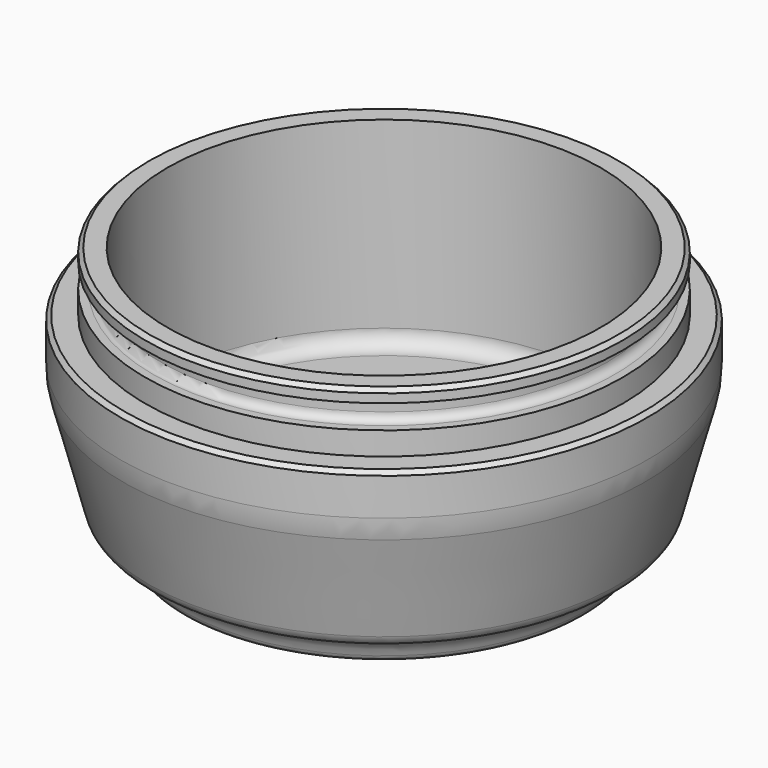
from build123d import *

# Parameters (mm, degrees)
F3_R    = 2
F4_R    = 1
F5_R    = 2
F8_R    = 10
F6_SIZE = 0.5
F9_SIZE = 0.5
F7_R    = 1


# Not quite as in the source:
# - a fillet or chamfer that OpenCascade refuses, or shapes differently, is made with other operations: its cross-section is extruded or revolved along the edge and cut away or added


with BuildPart() as f1:
    # F0 (on Front) → F1 (revolve)
    with BuildSketch(Plane.XZ):
        Polygon((0, -6.6736775178), (-27.25, -6.6736775178), (-27.25, 18.4263224822), (-30.05, 18.4263224822), (-30.05, 16.8263224822), (-28.05, 16.8263224822), (-28.05, 13.8263224822), (-30.05, 13.8263224822), (-30.05, 10.9263224822), (-33.2, 10.9263224822), (-33.2, 4.4263224822), (-29.2, -10.5736775178), (-25.2, -10.5736775178), (-25.2, -14.3736775178), (-22.2, -14.3736775178), (-20.5283898626, -10.1736775178), (0, -10.1736775178), align=None)
    revolve(axis=Axis((0, 0, -8.4236775178), (0, 0, 1)))

    # F2: fillet of radius 4 on 1 edges, made by hand

    # F2_s1 → F2_t2 (revolve)
    with BuildSketch(Plane.XZ):
        with BuildLine():
            ThreePointArc((-29.1949968711, -10.5736775178), (-26.4381871207, -11.6754021686), (-25.2, -14.3736775178))
            Line((-25.2, -14.3736775178), (-25.2, -10.5736775178))
            Line((-25.2, -10.5736775178), (-29.1949968711, -10.5736775178))
        make_face()
    revolve(axis=Axis((0, 0, -10.5736775178), (0, 0, 1)))

    # F3
    f3_edges = [f1.edges().sort_by_distance(p)[0] for p in [
        (27.25, 0, -6.673678),
    ]]
    fillet(f3_edges, radius=F3_R)

    # F4
    f4_edges = [f1.edges().sort_by_distance(p)[0] for p in [
        (25.2, 0, -14.373678),
    ]]
    fillet(f4_edges, radius=F4_R)

    # F5
    f5_edges = [f1.edges().sort_by_distance(p)[0] for p in [
        (29.2, 0, -10.573678),
    ]]
    fillet(f5_edges, radius=F5_R)

    # F8
    f8_edges = [f1.edges().sort_by_distance(p)[0] for p in [
        (33.2, 0, 4.426322),
    ]]
    fillet(f8_edges, radius=F8_R)

    # F6
    f6_edges = [f1.edges().sort_by_distance(p)[0] for p in [
        (30.05, 0, 18.426322),
    ]]
    chamfer(f6_edges, length=F6_SIZE)

    # F9
    f9_edges = [f1.edges().sort_by_distance(p)[0] for p in [
        (33.2, 0, 10.926322),
    ]]
    chamfer(f9_edges, length=F9_SIZE)

    # F7
    f7_edges = [f1.edges().sort_by_distance(p)[0] for p in [
        (28.05, 0, 16.826322),
        (28.05, 0, 13.826322),
    ]]
    fillet(f7_edges, radius=F7_R)


solid = f1.part
